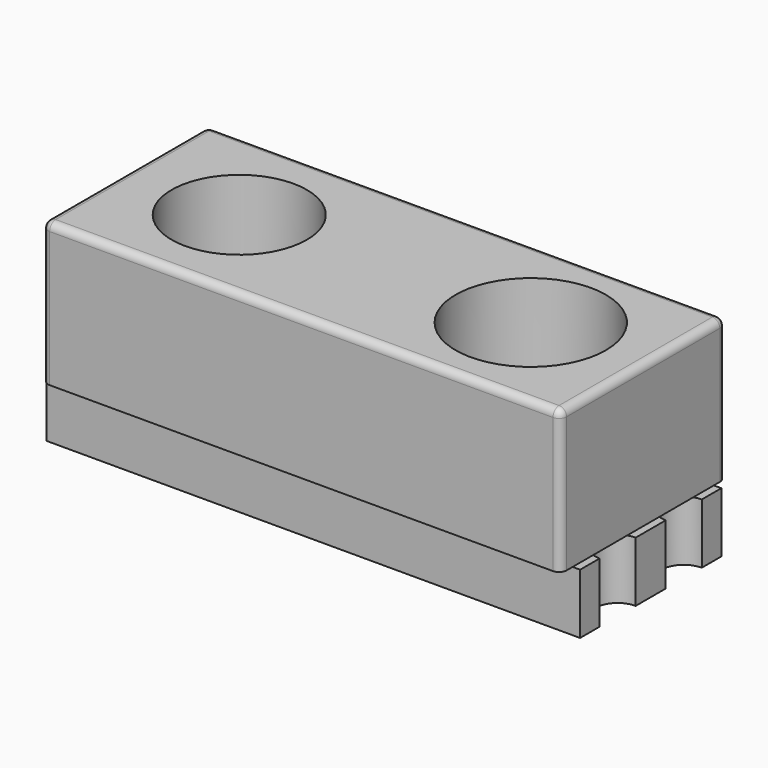
from build123d import *

# Parameters (mm, degrees)
F1_DEPTH = 0.8
F2_R     = 0.9
F2_R_2   = 1
F2_W     = 6.9
F2_H     = 0.2
F3_DEPTH = 1.9
F4_R     = 0.1


with BuildPart() as f1:
    # F0 (on Top) → F1 (new body)
    with BuildSketch(Plane.XY):
        with BuildLine():
            Line((0, 0.325), (0, 0))
            Line((0, 0), (7.1, 0))
            Line((7.1, 0), (7.1, 0.325))
            ThreePointArc((7.1, 0.325), (6.8, 0.625), (7.1, 0.925))
            Line((7.1, 0.925), (7.1, 1.425))
            ThreePointArc((7.1, 1.425), (6.8, 1.725), (7.1, 2.025))
            Line((7.1, 2.025), (7.1, 2.35))
            Line((7.1, 2.35), (0, 2.35))
            Line((0, 2.35), (0, 2.025))
            ThreePointArc((0, 2.025), (0.2121320344, 1.9371320344), (0.3, 1.725))
            ThreePointArc((0.3, 1.725), (0.2121320344, 1.5128679656), (0, 1.425))
            Line((0, 1.425), (0, 0.925))
            ThreePointArc((0, 0.925), (0.2121320344, 0.8371320344), (0.3, 0.625))
            ThreePointArc((0.3, 0.625), (0.2121320344, 0.4128679656), (0, 0.325))
        make_face()
    extrude(amount=F1_DEPTH)

    # F2 (on face) → F3 (join)
    with BuildSketch(Plane.XY.offset(0.8)):
        with BuildLine():
            Line((7, 2.35), (0.1, 2.35))
            Line((0.1, 2.35), (0.1, 2.0078427125))
            ThreePointArc((0.1, 2.0078427125), (0.3, 1.725), (0.1, 1.4421572875))
            Line((0.1, 1.4421572875), (0.1, 0.9078427125))
            ThreePointArc((0.1, 0.9078427125), (0.3, 0.625), (0.1, 0.3421572875))
            Line((0.1, 0.3421572875), (0.1, 0))
            Line((0.1, 0), (7, 0))
            Line((7, 0), (7, 0.3421572875))
            ThreePointArc((7, 0.3421572875), (6.8, 0.625), (7, 0.9078427125))
            Line((7, 0.9078427125), (7, 1.4421572875))
            ThreePointArc((7, 1.4421572875), (6.8, 1.725), (7, 2.0078427125))
            Line((7, 2.0078427125), (7, 2.35))
        make_face()
        with Locations((1.6234196955, 1.175)):
            Circle(F2_R, mode=Mode.SUBTRACT)
        with Locations((5.5034196955, 1.175)):
            Circle(F2_R_2, mode=Mode.SUBTRACT)
        with Locations((3.55, 2.45)):
            Rectangle(F2_W, F2_H)
        with Locations((3.55, -0.1)):
            Rectangle(F2_W, F2_H)
        with BuildLine():
            ThreePointArc((0.1, 0.3421572875), (0.3, 0.625), (0.1, 0.9078427125))
            Line((0.1, 0.9078427125), (0.1, 0.3421572875))
        make_face()
        with BuildLine():
            ThreePointArc((0.1, 1.4421572875), (0.3, 1.725), (0.1, 2.0078427125))
            Line((0.1, 2.0078427125), (0.1, 1.4421572875))
        make_face()
        with BuildLine():
            Line((7, 1.4421572875), (7, 2.0078427125))
            ThreePointArc((7, 2.0078427125), (6.8, 1.725), (7, 1.4421572875))
        make_face()
        with BuildLine():
            Line((7, 0.3421572875), (7, 0.9078427125))
            ThreePointArc((7, 0.9078427125), (6.8, 0.625), (7, 0.3421572875))
        make_face()
    extrude(amount=F3_DEPTH)

    # F4
    f4_edges = [f1.edges().sort_by_distance(p)[0] for p in [
        (0.1, 1.175, 2.7),
        (0.1, -0.2, 1.75),
        (0.1, 2.55, 1.75),
        (7, -0.2, 1.75),
        (7, 2.55, 1.75),
        (3.55, 2.55, 2.7),
        (3.55, -0.2, 2.7),
        (7, 1.175, 2.7),
    ]]
    fillet(f4_edges, radius=F4_R)


solid = f1.part
